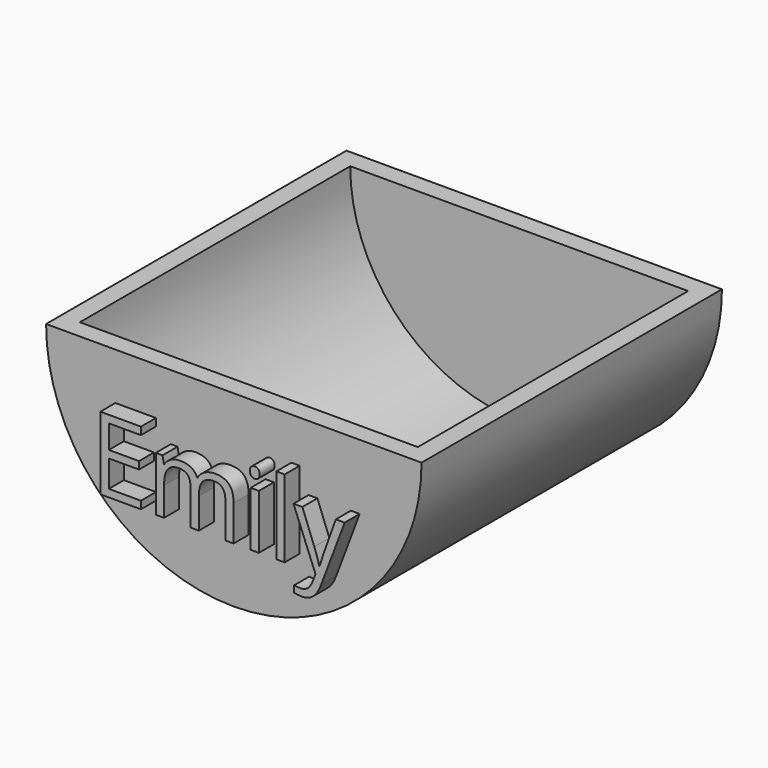
from build123d import *

# Parameters (mm, degrees)
F1_DEPTH     = 50.8
F2_T         = -2.54
F3_TEXT_SIZE = 13.7892351227
F4_DEPTH     = 2.54


# Not quite as in the source:
# - Text() gives the source's letters only with a copy of the font that has no kerning and outlines rounded to 1/6400 em; it was checked with that copy


with BuildPart() as f1:
    # F0 (on Front) → F1 (new body)
    with BuildSketch(Plane.XZ):
        with BuildLine():
            Line((25.4, 0), (0, 0))
            Line((0, 0), (0, -25.4))
            ThreePointArc((0, -25.4), (17.9605122421, -17.9605122421), (25.4, 0))
        make_face()
        with BuildLine():
            Line((0, -25.4), (0, 0))
            Line((0, 0), (-25.4, 0))
            ThreePointArc((-25.4, 0), (-17.9605122421, -17.9605122421), (0, -25.4))
        make_face()
    extrude(amount=F1_DEPTH)

    # F2
    f2_openings = [f1.faces().sort_by_distance(p)[0] for p in [
        (0, -25.4, 0),
    ]]
    offset(amount=F2_T, openings=f2_openings)

    # F3 (on face) → F4 (join)
    with BuildSketch(Plane.XZ.offset(50.8)):
        with Locations((-17.3744335771, -16.2064060569)):
            Text('Emily', F3_TEXT_SIZE, font='Open Sans', text_align=(TextAlign.LEFT, TextAlign.BOTTOM))
    extrude(amount=F4_DEPTH)


solid = f1.part
